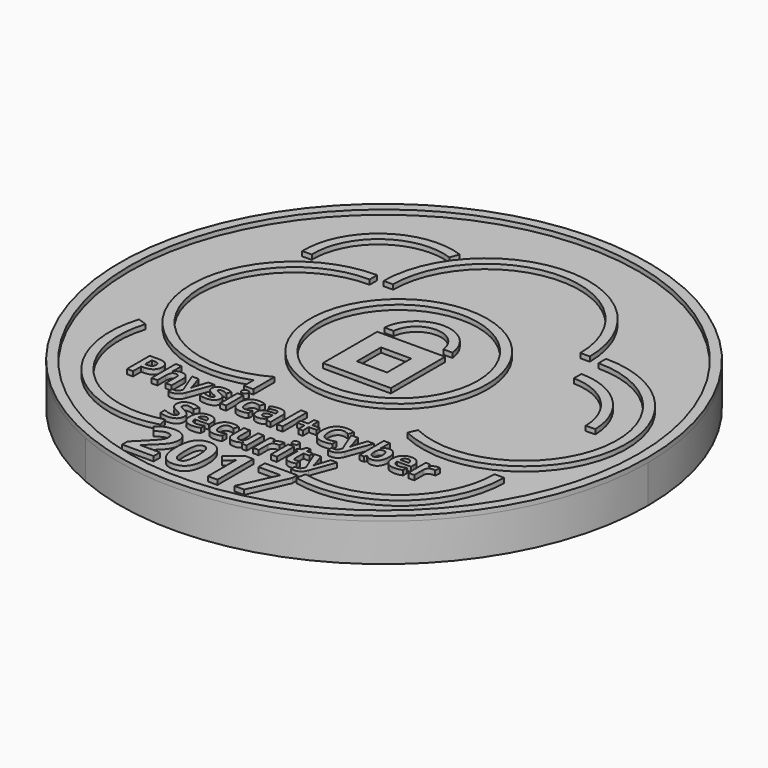
from build123d import *
from build123d import SkipClean  # not in build123d's __all__

# Parameters (mm, degrees)
F1_DEPTH       = 3.175
F2_R           = 22.225
F2_R_2         = 21.43125
F3_DEPTH       = 0.396875
F4_W           = 5.715
F4_H           = 5.715
F4_W_2         = 2.54
F4_H_2         = 2.54
F5_DEPTH       = 0.396875
F6_TEXT_SIZE   = 3.3517525773
F6_TEXT_SIZE_2 = 3.3517416667
F6_TEXT_SIZE_3 = 5.2916666667
F7_DEPTH       = 0.396875
F9_R           = 7.46125
F9_R_2         = 6.6675
F10_DEPTH      = 0.396875


# Not quite as in the source:
# - after a boolean that leaves OpenCascade's solid faulty, fix() repairs it
# - Text() gives the source's letters only with a copy of the font that has no kerning and outlines rounded to 1/6400 em; it was checked with that copy


with BuildPart() as f1:
    # F0 (on Top) → F1 (new body)
    with BuildSketch(Plane.XY):
        with BuildLine():
            ThreePointArc((-8.8056988654, -20.4061336978), (-13.024927703, -7.0845045011), (-21.9154725052, 3.6963076))
            ThreePointArc((-21.9154725052, 3.6963076), (-19.5238190865, -10.6193744296), (-8.8056988654, -20.4061336978))
        make_face()
        with BuildLine():
            ThreePointArc((-8.8056988654, -20.4061336978), (12.211551247, -18.5695622227), (22.225, 0))
            ThreePointArc((22.225, 0), (1.8546224106, 22.1474829431), (-21.9154725052, 3.6963076))
            ThreePointArc((-21.9154725052, 3.6963076), (-13.024927703, -7.0845045011), (-8.8056988654, -20.4061336978))
        make_face()
    extrude(amount=-F1_DEPTH)

    # F2 (on Top) → F3 (join)
    with BuildSketch(Plane.XY):
        Circle(F2_R)
        Circle(F2_R_2, mode=Mode.SUBTRACT)
    with SkipClean():  # cleaning this boolean's faces spoils the solid; the shape is the same uncleaned
        extrude(amount=F3_DEPTH)

    # F4 (on Top) → F5 (join)
    with BuildSketch(Plane.XY):
        Rectangle(F4_W, F4_H)
        Rectangle(F4_W_2, F4_H_2, mode=Mode.SUBTRACT)
        with BuildLine():
            Line((2.0955, 3.6195), (2.8575, 3.6195))
            ThreePointArc((2.8575, 3.6195), (0, 6.2563072639), (-2.8575, 3.6195))
            Line((-2.8575, 3.6195), (-2.0955, 3.6195))
            ThreePointArc((-2.0955, 3.6195), (0, 5.5003360277), (2.0955, 3.6195))
        make_face()
    extrude(amount=F5_DEPTH)

    add(f1.part.fix(), mode=Mode.REPLACE)

    # F6 (on Top) → F7 (join)
    with BuildSketch(Plane.XY):
        with Locations((-12.7, -11.5572618557)):
            Text('Physical+Cyber', F6_TEXT_SIZE, font='Open Sans', font_style=FontStyle.BOLD, text_align=(TextAlign.LEFT, TextAlign.BOTTOM))
        with Locations((-6.93810525, -15.1611408557)):
            Text('Security', F6_TEXT_SIZE_2, font='Open Sans', font_style=FontStyle.BOLD, text_align=(TextAlign.LEFT, TextAlign.BOTTOM))
        with Locations((-6.1284114583, -20.1617658557)):
            Text('2017', F6_TEXT_SIZE_3, font='Open Sans', font_style=FontStyle.BOLD, text_align=(TextAlign.LEFT, TextAlign.BOTTOM))
    extrude(amount=F7_DEPTH)

    # F9 (on Top) → F10 (join)
    with BuildSketch(Plane.XY):
        with Locations((0, 1.5449698431)):
            Circle(F9_R)
        with Locations((0, 1.5449698431)):
            Circle(F9_R_2, mode=Mode.SUBTRACT)
        with BuildLine():
            ThreePointArc((-6.2640812248, 8.7699014693), (1.5688695108, 16.6018772131), (9.4657531008, 8.8343685493))
            Line((9.4657531008, 8.8343685493), (10.2594418851, 8.8442263519))
            ThreePointArc((10.2594418851, 8.8442263519), (1.5656164368, 17.3956205469), (-7.0578241475, 8.7732533492))
            Line((-7.0578241475, 8.7732533492), (-6.2640812248, 8.7699014693))
        make_face()
        with BuildLine():
            ThreePointArc((-4.1074021719, -6.3834940083), (-15.5804862414, -1.4753258737), (-7.9020801932, 8.3615360782))
            Line((-7.9020801932, 8.3615360782), (-7.8967955751, 9.155268486))
            ThreePointArc((-7.8967955751, 9.155268486), (-16.4878188027, -1.0361025059), (-4.9011521719, -7.6254028617))
            Line((-4.9011521719, -7.6254028617), (-4.9011521719, -8.62644054))
            Line((-4.9011521719, -8.62644054), (-4.1074021719, -8.62644054))
            Line((-4.1074021719, -8.62644054), (-4.1074021719, -6.3834940083))
        make_face()
        with BuildLine():
            ThreePointArc((-5.94648486, -15.6169785187), (-13.6110446514, -13.5353809318), (-15.4331782833, -5.8050281368))
            Line((-15.4331782833, -5.8050281368), (-16.1901574778, -5.5662362576))
            ThreePointArc((-16.1901574778, -5.5662362576), (-14.1816891259, -14.087109077), (-5.7333374233, -16.3815746426))
            Line((-5.7333374233, -16.3815746426), (-5.94648486, -15.6169785187))
        make_face()
        with BuildLine():
            ThreePointArc((15.8507805318, -8.1708543003), (12.8422727132, -14.3562987448), (6.1485688202, -15.9390717745))
            Line((6.1485688202, -15.9390717745), (5.9825126086, -16.7152575751))
            ThreePointArc((5.9825126086, -16.7152575751), (13.3383754618, -14.9759124352), (16.644492861, -8.1785874045))
            Line((16.644492861, -8.1785874045), (15.8507805318, -8.1708543003))
        make_face()
        with BuildLine():
            ThreePointArc((11.3767180592, 5.7565816678), (14.7582622479, 4.3381334803), (16.2086989731, 0.9701860836))
            Line((16.2086989731, 0.9701860836), (17.0022359099, 0.9885760912))
            ThreePointArc((17.0022359099, 0.9885760912), (15.316861918, 4.9020532184), (11.3875856323, 6.550257268))
            Line((11.3875856323, 6.550257268), (11.3767180592, 5.7565816678))
        make_face()
        with BuildLine():
            ThreePointArc((11.304073967, 8.4475371987), (18.9248980247, -1.0438867527), (7.997283712, -6.4059137367))
            Line((7.997283712, -6.4059137367), (7.6596225792, -7.1242618569))
            ThreePointArc((7.6596225792, -7.1242618569), (19.6996799115, -1.2163746954), (11.3030476779, 9.2412865352))
            Line((11.3030476779, 9.2412865352), (11.304073967, 8.4475371987))
        make_face()
        with BuildLine():
            ThreePointArc((-13.0916433409, 8.7592359632), (-10.8401113296, 13.3596624922), (-5.7702260092, 14.0873873606))
            Line((-5.7702260092, 14.0873873606), (-5.5025462486, 14.8346400677))
            ThreePointArc((-5.5025462486, 14.8346400677), (-11.3071723572, 14.0014514443), (-13.8850021641, 8.7343192998))
            Line((-13.8850021641, 8.7343192998), (-13.0916433409, 8.7592359632))
        make_face()
    extrude(amount=F10_DEPTH)


solid = f1.part
